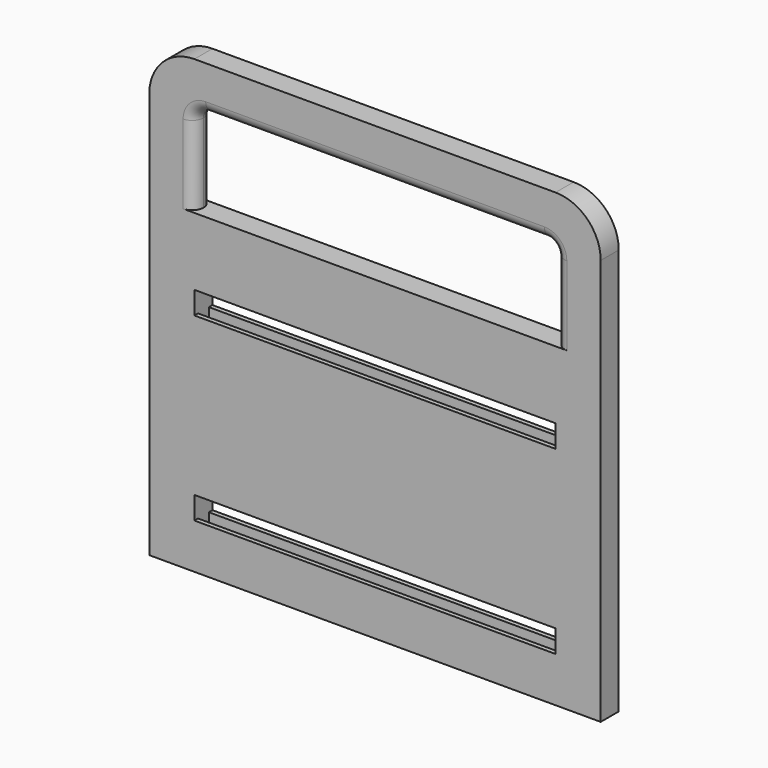
from build123d import *

# Parameters (mm, degrees)
F0_W          = 160
F0_H          = 10
F0_H_2        = 40
F1_DEPTH      = 5
F1_DEPTH_BACK = 5
F2_F1_R       = 5
F2_F2_R       = 4.9999
F3_R          = 20
F4_W          = 160
F4_H          = 6
F5_DEPTH      = 6
F6_W          = 160
F6_H          = 6
F7_DEPTH      = 6


# Not quite as in the source:
# - a fillet or chamfer is up to 0.001 mm smaller than in the source, because OpenCascade refuses the exact size


with BuildPart() as f1:
    # F0 (on Front) → F1 (new body, two sides)
    with BuildSketch(Plane.XZ) as f1_sk:
        Polygon((-100, 0), (0, 0), (100, 0), (100, 200), (0, 200), (-100, 200), align=None)
        with Locations((0, 25)):
            Rectangle(F0_W, F0_H, mode=Mode.SUBTRACT)
        with Locations((0, 105)):
            Rectangle(F0_W, F0_H, mode=Mode.SUBTRACT)
        with Locations((0, 160)):
            Rectangle(F0_W, F0_H_2, mode=Mode.SUBTRACT)
    extrude(amount=F1_DEPTH)
    extrude(f1_sk.sketch, amount=-F1_DEPTH_BACK)

    # F2: fillet of radius 5 on 4 edges, made by hand

    # F2_f1
    f2_f1_edges = [f1.edges().sort_by_distance(p)[0] for p in [
        (80, 0, 180),
        (-80, 0, 180),
    ]]
    fillet(f2_f1_edges, radius=F2_F1_R)

    # F2_f2 (radius 5 in the source; OpenCascade refuses exactly that, so slightly less here)
    f2_f2_edges = [f1.edges().sort_by_distance(p)[0] for p in [
        (0, -5, 180),
        (0, 5, 180),
        (-78.5355339059, 5, 178.5355339059),
        (78.5355339059, 5, 178.5355339059),
        (-78.5355339059, -5, 178.5355339059),
        (78.5355339059, -5, 178.5355339059),
    ]]
    fillet(f2_f2_edges, radius=F2_F2_R)

    # F3
    f3_edges = [f1.edges().sort_by_distance(p)[0] for p in [
        (-100, 0, 200),
        (100, 0, 200),
    ]]
    fillet(f3_edges, radius=F3_R)

    # F4 (on face) → F5 (cut)
    with BuildSketch(Plane.XY.offset(20)):
        Rectangle(F4_W, F4_H)
    extrude(amount=-F5_DEPTH, mode=Mode.SUBTRACT)

    # F6 (on face) → F7 (cut)
    with BuildSketch(Plane.XY.offset(100)):
        Rectangle(F6_W, F6_H)
    extrude(amount=-F7_DEPTH, mode=Mode.SUBTRACT)


solid = f1.part
